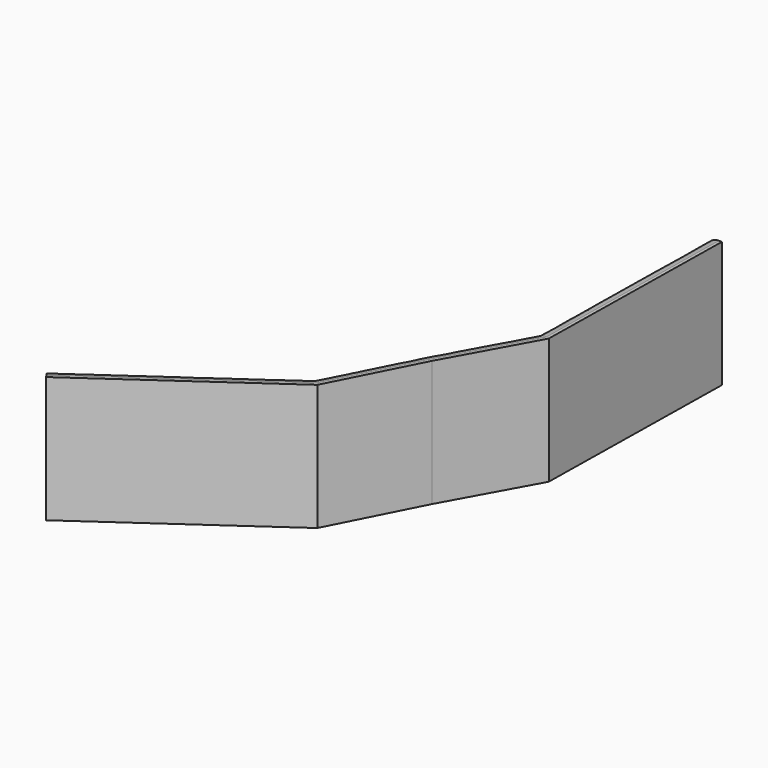
from build123d import *

# Parameters (mm, degrees)
F5_D = 100
F7_D = 100


# Not quite as in the source:
# - a feature names something its author has since deleted; it is built from what else it names


with BuildPart() as f2:
    # F2: sweep along a path in F1
    with BuildLine(Plane.XY) as f2_path:
        Line((-107.3189526796, -226.6205847263), (-115.9728169441, -761.2517476082))
        Line((-115.9728169441, -761.2517476082), (-413.3533239365, -1301.2853860855))
    # F0 (on Front) → F2 (sweep)
    with BuildSketch(Plane.XZ):
        with BuildLine():
            Line((-836.5186393261, 158.2419019938), (-836.5186393261, 148.2419019938))
            Line((-836.5186393261, 148.2419019938), (-436.5186393261, 148.2419019938))
            Line((-436.5186393261, 148.2419019938), (-436.5186393261, 548.2419019938))
            Line((-436.5186393261, 548.2419019938), (-446.5186393261, 548.2419019938))
            ThreePointArc((-446.5186393261, 548.2419019938), (-474.8029105736, 536.5261732412), (-486.5186393261, 508.2419019938))
            Line((-486.5186393261, 508.2419019938), (-486.5186393261, 248.2419019938))
            ThreePointArc((-486.5186393261, 248.2419019938), (-501.1633002668, 212.8865629344), (-536.5186393261, 198.2419019938))
            Line((-536.5186393261, 198.2419019938), (-796.5186393261, 198.2419019938))
            ThreePointArc((-796.5186393261, 198.2419019938), (-824.8029105736, 186.5261732412), (-836.5186393261, 158.2419019938))
        make_face()
    sweep(path=f2_path.line, transition=Transition.RIGHT)

    # F3: F2 across face


with BuildPart() as f2_1:
    add(f2.part)
    add(f2.part.mirror(Plane(origin=(-700.4191524375, -892.7521403639, 263.9571660189), x_dir=(0.8836600113, -0.4681292389, 0), z_dir=(-0.4681292389, -0.8836600113, 0))))

    # F5 (through all)
    with Locations(Plane.XY.offset(198.2419019938)):
        with Locations((-667.7702069283, -149.9368995428)):
            Hole(F5_D / 2)

    # F7 (through all)
    with Locations(Plane.XY.offset(198.2419019938)):
        with Locations((-1321.2910347152, -1389.5985503476)):
            Hole(F7_D / 2)


solid = f2_1.part
